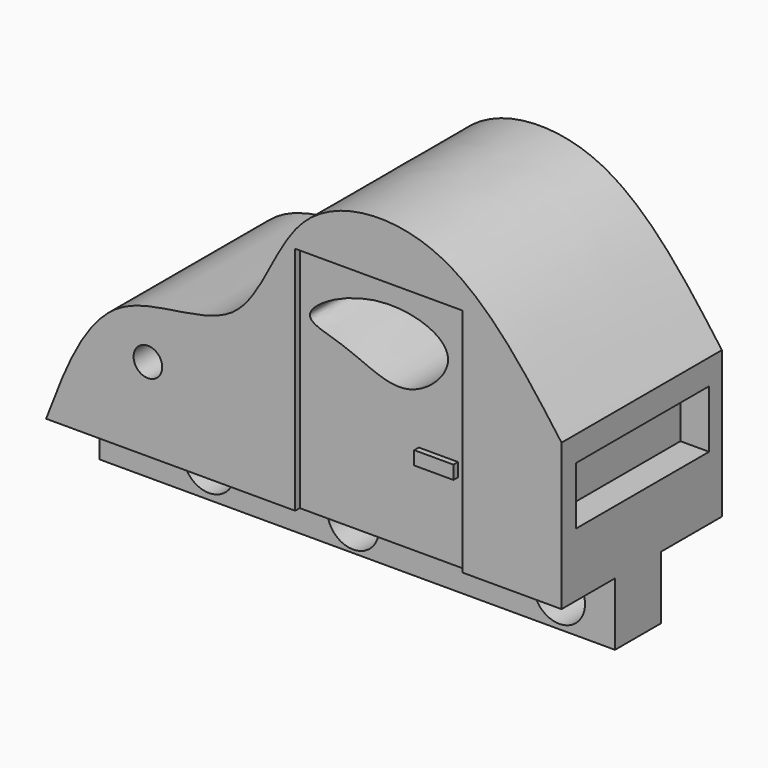
from build123d import *

# Parameters (mm, degrees)
F0_W      = 2286
F0_H      = 889
F1_DEPTH  = 1778
F3_DEPTH  = 889
F5_DEPTH  = 889
F6_W      = 736.6
F6_H      = 256.0062574527
F7_DEPTH  = 127
F8_W      = 2286
F8_H      = 254.1629374027
F9_DEPTH  = 279.4
F10_R     = 114.3
F11_DEPTH = 381
F12_R     = 114.3
F13_DEPTH = 381
F14_W     = 741.9006824493
F14_H     = 1022.9654312134
F15_DEPTH = 25.4
F16_W     = 173.9646
F16_H     = 59.8678
F17_DEPTH = 25.4
F18_R     = 63.5
F19_DEPTH = 889
F20_R     = 114.3
F21_DEPTH = 381


# Not quite as in the source:
# - a feature names something its author has since deleted; it is built from what else it names


with BuildPart() as f1:
    # F0 (on Top) → F1 (new body)
    with BuildSketch(Plane.XY):
        with Locations((515.3457043618, 148.0594710579)):
            Rectangle(F0_W, F0_H)
    extrude(amount=F1_DEPTH)

    # F2 (on face) → F3 (cut)
    with BuildSketch(Plane.XZ.offset(296.4405289421)):
        with BuildLine():
            Line((-627.6542956382, 1778), (-627.6542956382, 0))
            add(Edge.make_bspline(
                [(-627.6542956382, 0), (-541.4336594546, 228.5495208712), (-378.466489085, 660.5350681174), (292.3103575218, 559.8639582491), (430.6892955486, 1252.6841744519), (1165.5216956238, 1322.9601242052), (1484.4969995752, 887.4267608137), (1658.3457043618, 650.0512957573)],
                knots=[0, 0, 0, 0, 0.2047131286, 0.3869319548, 0.5782611503, 0.7701428547, 1, 1, 1, 1], degree=3))
            Line((1658.3457043618, 650.0512957573), (1658.3457043618, 1778))
            Line((1658.3457043618, 1778), (-627.6542956382, 1778))
        make_face()
    extrude(amount=-F3_DEPTH, mode=Mode.SUBTRACT)

    # F4 (on face) → F5 (cut)
    with BuildSketch(Plane.XZ.offset(296.4405289421)):
        with BuildLine():
            add(Edge.make_bspline(
                [(522.1207141876, 767.1055197716), (519.7513293275, 813.9735385683), (815.0612749868, 989.7990248624), (1253.0272817349, 842.7583173423), (951.3919468713, 543.5567329303), (707.3552544441, 704.1588627621), (523.8330636603, 733.2341008126), (522.1207141876, 767.1055197716)],
                knots=[0, 0, 0, 0, 0.2201911252, 0.4422931214, 0.6337376897, 0.8408683353, 1, 1, 1, 1], degree=3))
        make_face()
    extrude(amount=-F5_DEPTH, mode=Mode.SUBTRACT)

    # F6 (on face) → F7 (cut)
    with BuildSketch(Plane.YZ.offset(1658.3457043618)):
        with Locations((153.1417667866, 410.0026041269)):
            Rectangle(F6_W, F6_H)
    extrude(amount=-F7_DEPTH, mode=Mode.SUBTRACT)

    # F8 (on face) → F9 (join)
    with BuildSketch(Plane(origin=(0, 0, 0), x_dir=(1, 0, 0), z_dir=(0, 0, -1))):
        with Locations((515.3457043618, -127.0814687014)):
            Rectangle(F8_W, F8_H)
    extrude(amount=F9_DEPTH)

    # F10 (on face) → F11 (cut)
    with BuildSketch(Plane(origin=(0, 254.1629374027, 0), x_dir=(-1, 0, 0), z_dir=(0, 1, 0))):
        with Locations((-1411.1014604568, -143.9275145531)):
            Circle(F10_R)
    extrude(amount=-F11_DEPTH, mode=Mode.SUBTRACT)

    # F12 (on face) → F13 (cut)
    with BuildSketch(Plane.XZ):
        with Locations((496.906042099, -151.1470973492)):
            Circle(F12_R)
    extrude(amount=-F13_DEPTH, mode=Mode.SUBTRACT)

    # F14 (on face) → F15 (cut)
    with BuildSketch(Plane.XZ.offset(296.4405289421)):
        with Locations((848.0150699615, 511.4827156067)):
            Rectangle(F14_W, F14_H)
        with BuildLine():
            add(Edge.make_bspline(
                [(522.1207141876, 767.1055197716), (519.7513293275, 813.9735385683), (815.0612749868, 989.7990248624), (1253.0272817349, 842.7583173423), (951.3919468713, 543.5567329303), (707.3552544441, 704.1588627621), (523.8330636603, 733.2341008126), (522.1207141876, 767.1055197716)],
                knots=[0, 0, 0, 0, 0.2201911252, 0.4422931214, 0.6337376897, 0.8408683353, 1, 1, 1, 1], degree=3))
        make_face(mode=Mode.SUBTRACT)
    extrude(amount=-F15_DEPTH, mode=Mode.SUBTRACT)

    # F16 (on face) → F17 (join)
    with BuildSketch(Plane.XZ.offset(271.0405289421)):
        with Locations((1091.9465520813, 378.4035745872)):
            Rectangle(F16_W, F16_H)
    extrude(amount=F17_DEPTH)

    # F18 (on face) → F19 (cut)
    with BuildSketch(Plane.XZ.offset(296.4405289421)):
        with Locations((-176.0771423578, 368.7046468258)):
            Circle(F18_R)
    extrude(amount=-F19_DEPTH, mode=Mode.SUBTRACT)

    # F20 (on face) → F21 (cut)
    with BuildSketch(Plane(origin=(0, 254.1629374027, 0), x_dir=(-1, 0, 0), z_dir=(0, 1, 0))):
        with Locations((142.4564868212, -138.3589059114)):
            Circle(F20_R)
    extrude(amount=-F21_DEPTH, mode=Mode.SUBTRACT)


solid = f1.part
